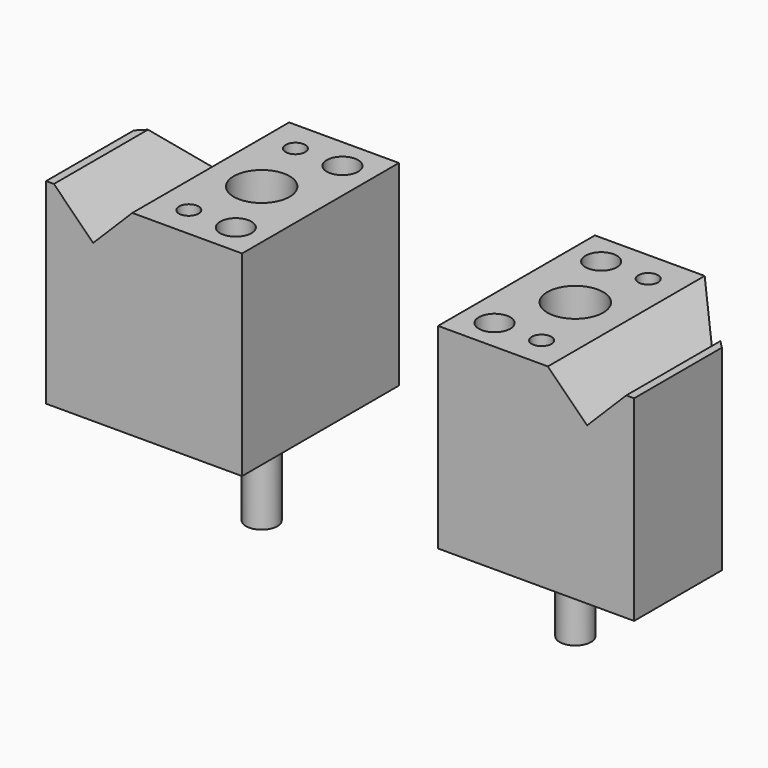
from build123d import *

# Parameters (mm, degrees)
F0_W           = 50
F0_H           = 50
F1_DEPTH       = 50
F3_DEPTH       = 50.001
F4_R           = 4
F5_DEPTH       = 25
F7_D           = 5
F7_DEPTH       = 20
F7_TIP         = 1.5021515476
F8_D           = 7.4
F8_DEPTH       = 60
F8_CBORE_D     = 14.25
F8_CBORE_DEPTH = 8
F8_TIP         = 2.2231842904
F9_R           = 4
F10_DEPTH      = 25
F12_DEPTH      = 75.001


# Not quite as in the source:
# - a feature names something its author has since deleted; it is built from what else it names


with BuildPart() as f1:
    # F0 (on Top) → F1 (new body)
    with BuildSketch(Plane.XY):
        Rectangle(F0_W, F0_H)
    extrude(amount=F1_DEPTH)

    # F2 (on face) → F3 (cut, through all)
    with BuildSketch(Plane.XZ.offset(25)):
        Polygon((13, 40), (23, 50), (3, 50), align=None)
    extrude(amount=-F3_DEPTH, mode=Mode.SUBTRACT)

    # F4 (on face) → F5 (cut)
    with BuildSketch(Plane.XY.offset(50)):
        with Locations((-17, 17)):
            Circle(F4_R)
        with Locations((-17, -17)):
            Circle(F4_R)
    extrude(amount=-F5_DEPTH, mode=Mode.SUBTRACT)

    # F7
    with Locations(Plane.XY.offset(50)):
        with Locations((-5, -17), (-5, 17)):
            Hole(F7_D / 2, depth=F7_DEPTH)
            with Locations((0, 0, -(F7_DEPTH + F7_TIP / 2))):  # 118° drill point
                Cone(0, F7_D / 2, F7_TIP, mode=Mode.SUBTRACT)

    # F8
    with Locations(Plane.XY.offset(50)):
        with Locations((-10, 0)):
            CounterBoreHole(F8_D / 2, F8_CBORE_D / 2, F8_CBORE_DEPTH, depth=F8_DEPTH)
            with Locations((0, 0, -(F8_DEPTH + F8_TIP / 2))):  # 118° drill point
                Cone(0, F8_D / 2, F8_TIP, mode=Mode.SUBTRACT)

    # F9 (on face) → F10 (join)
    with BuildSketch(Plane(origin=(0, 0, 0), x_dir=(1, 0, 0), z_dir=(0, 0, -1))):
        with Locations((-10, 0)):
            Circle(F9_R)
    extrude(amount=F10_DEPTH)

    # F11 (on face) → F12 (cut, through all)
    with BuildSketch(Plane.XY.offset(50)):
        Polygon((28, 25), (3, 25), (28, 0), align=None)
    extrude(amount=-F12_DEPTH, mode=Mode.SUBTRACT)


with BuildPart() as f13_1:
    # F13: instance of F1
    add(f1.part.mirror(Plane(origin=(-25, 0, 25), x_dir=(0, -1, 0), z_dir=(-1, 0, 0))))


with BuildPart() as f13_1_1:
    # F14: moved
    add(f13_1.part.moved(Location((-50, 0, 0))))


solid = Compound([f1.part, f13_1_1.part])
